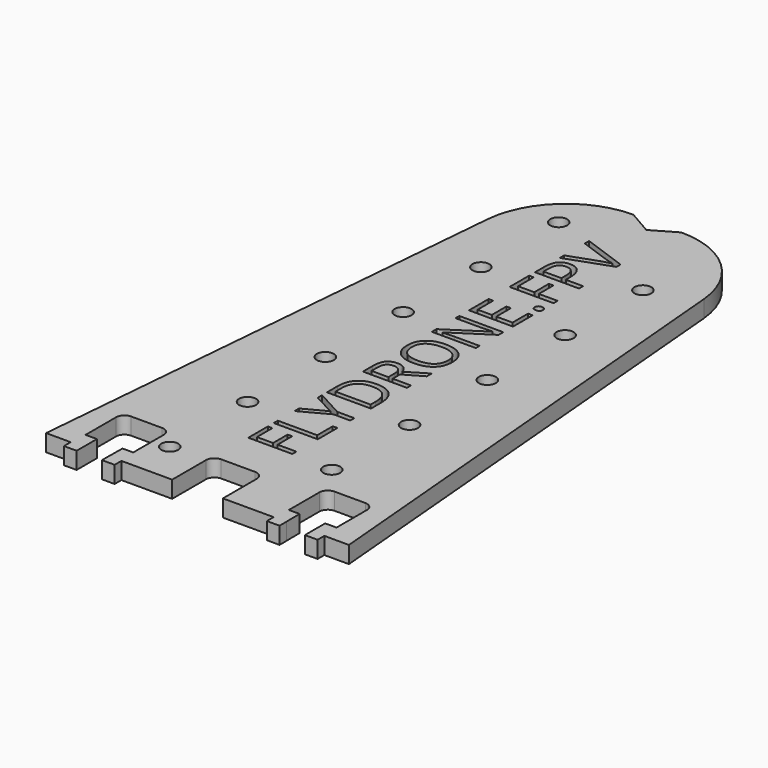
from build123d import *

# Parameters (mm, degrees)
F0_R         = 1
F1_DEPTH     = 2
F2_TEXT_SIZE = 7.292155104
F3_DEPTH     = 25


# Not quite as in the source:
# - Text() gives the source's letters only with a copy of the font that has no kerning and outlines rounded to 1/6400 em; it was checked with that copy


with BuildPart() as f1:
    # F0 (on Top) → F1 (new body)
    with BuildSketch(Plane.XY):
        with BuildLine():
            Line((17.9130434783, -33.5), (12.7942351162, 25.3662961636))
            ThreePointArc((12.7942351162, 25.3662961636), (9.5896779438, 31.8709891343), (2.8318292342, 34.5))
            Line((2.8318292342, 34.5), (0, 32.8609384596))
            Line((0, 32.8609384596), (-2.8318292342, 34.5))
            ThreePointArc((-2.8318292342, 34.5), (-9.5896779438, 31.8709891343), (-12.7942351162, 25.3662961636))
            Line((-12.7942351162, 25.3662961636), (-17.9130434783, -33.5))
            Line((-17.9130434783, -33.5), (-15, -33.5))
            Line((-15, -33.5), (-15, -34.5))
            Line((-15, -34.5), (-13.5, -34.5))
            Line((-13.5, -34.5), (-13.5, -33.5))
            Line((-13.5, -33.5), (-13.5, -31.5))
            Line((-13.5, -31.5), (-14.84164875, -31.5))
            Line((-14.84164875, -31.5), (-14.84164875, -27))
            ThreePointArc((-14.84164875, -27), (-14.5487555312, -26.2928932188), (-13.84164875, -26))
            Line((-13.84164875, -26), (-10.2081930488, -26))
            ThreePointArc((-10.2081930488, -26), (-9.5010862676, -26.2928932188), (-9.2081930488, -27))
            Line((-9.2081930488, -27), (-9.2081930488, -31.5))
            Line((-9.2081930488, -31.5), (-10.4703691453, -31.5))
            Line((-10.4703691453, -31.5), (-10.5, -33.5))
            Line((-10.5, -33.5), (-10.5, -34.5))
            Line((-10.5, -34.5), (-9, -34.5))
            Line((-9, -34.5), (-9, -33.5))
            Line((-9, -33.5), (-3, -33.5))
            Line((-3, -33.5), (-3, -31.5))
            Line((-3, -31.5), (-3, -28.5))
            ThreePointArc((-3, -28.5), (-2.7071067812, -27.7928932188), (-2, -27.5))
            Line((-2, -27.5), (-1, -27.5))
            Line((-1, -27.5), (1, -27.5))
            Line((1, -27.5), (2, -27.5))
            ThreePointArc((2, -27.5), (2.7071067812, -27.7928932188), (3, -28.5))
            Line((3, -28.5), (3, -31.5))
            Line((3, -31.5), (3, -33.5))
            Line((3, -33.5), (9, -33.5))
            Line((9, -33.5), (9, -34.5))
            Line((9, -34.5), (10.5, -34.5))
            Line((10.5, -34.5), (10.5, -33.5))
            Line((10.5, -33.5), (10.4703691453, -31.5))
            Line((10.4703691453, -31.5), (9.2081930488, -31.5))
            Line((9.2081930488, -31.5), (9.2081930488, -27))
            ThreePointArc((9.2081930488, -27), (9.5010862676, -26.2928932188), (10.2081930488, -26))
            Line((10.2081930488, -26), (13.84164875, -26))
            ThreePointArc((13.84164875, -26), (14.5487555312, -26.2928932188), (14.84164875, -27))
            Line((14.84164875, -27), (14.84164875, -31.5))
            Line((14.84164875, -31.5), (13.5, -31.5))
            Line((13.5, -31.5), (13.5, -33.5))
            Line((13.5, -33.5), (13.5, -34.5))
            Line((13.5, -34.5), (15, -34.5))
            Line((15, -34.5), (15, -33.5))
            Line((15, -33.5), (17.9130434783, -33.5))
        make_face()
        with Locations((-7.2821952552, -28.5)):
            Circle(F0_R, mode=Mode.SUBTRACT)
        with Locations((-7.2821952552, -17)):
            Circle(F0_R, mode=Mode.SUBTRACT)
        with Locations((-7.2821952552, -5.5)):
            Circle(F0_R, mode=Mode.SUBTRACT)
        with Locations((7.2821952552, -22.75)):
            Circle(F0_R, mode=Mode.SUBTRACT)
        with Locations((7.2821952552, -11.25)):
            Circle(F0_R, mode=Mode.SUBTRACT)
        with Locations((-7.2821952552, 6)):
            Circle(F0_R, mode=Mode.SUBTRACT)
        with Locations((-7.2821952552, 17.5)):
            Circle(F0_R, mode=Mode.SUBTRACT)
        with Locations((-7.2821952552, 29)):
            Circle(F0_R, mode=Mode.SUBTRACT)
        with Locations((7.2821952552, 0.25)):
            Circle(F0_R, mode=Mode.SUBTRACT)
        with Locations((7.2821952552, 11.75)):
            Circle(F0_R, mode=Mode.SUBTRACT)
        with Locations((7.2821952552, 23.25)):
            Circle(F0_R, mode=Mode.SUBTRACT)
    extrude(amount=F1_DEPTH)

    # F2 (on face) → F3 (cut)
    with BuildSketch(Plane.XY.offset(2)):
        with Locations(Location((2.460065938, -23.2749293487), (0, 0, 90))):
            Text('FLYDRONE.FPV', F2_TEXT_SIZE, font='Open Sans', text_align=(TextAlign.LEFT, TextAlign.BOTTOM))
    extrude(amount=-F3_DEPTH, mode=Mode.SUBTRACT)


solid = f1.part
